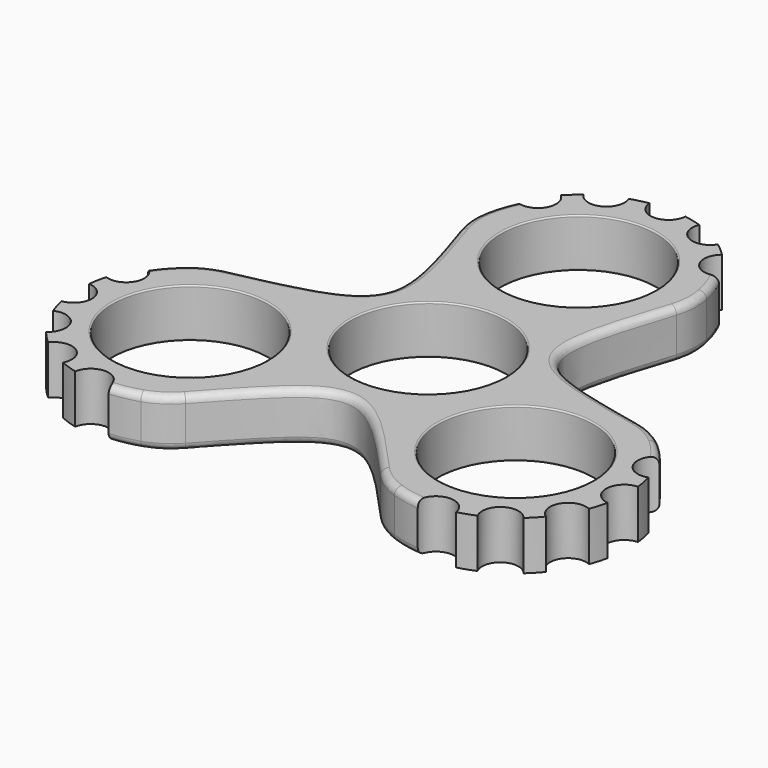
from build123d import *

# Parameters (mm, degrees)
F0_R     = 11.15
F2_DEPTH = 7
F3_COUNT = 3
F4_R     = 10
F5_R     = 1
F6_R     = 0.2


with BuildPart() as f2:
    # F0 (on Top) → F2 (new body)
    with BuildSketch(Plane.XY):
        with BuildLine():
            add(Edge.make_bspline(
                [(16.15, 27), (9.1228665673, 5.2670894684), (9.1238828606, 5.2676762256), (31.4576859022, 0.4863102711)],
                knots=[0, 0, 0, 0, 30.6153718044, 30.6153718044, 30.6153718044, 30.6153718044], degree=3))
            ThreePointArc((16.15, 27), (15.743464838, 30.6008075335), (14.544326329, 34.0203327297))
            ThreePointArc((14.544326329, 34.0203327297), (11.0995102001, 34.7719607126), (11.5714074372, 38.2661009192))
            ThreePointArc((11.5714074372, 38.2661009192), (10.6484349139, 39.1422128908), (9.6593461127, 39.9429336966))
            ThreePointArc((9.6593461127, 39.9429336966), (6.2566937093, 39.0189967896), (5.0618572759, 42.3362349004))
            ThreePointArc((5.0618572759, 42.3362349004), (3.8386271611, 42.6871744275), (2.5915629578, 42.9407120743))
            ThreePointArc((2.5915629578, 42.9407120743), (0, 40.55), (-2.5915629578, 42.9407120743))
            ThreePointArc((-2.5915629578, 42.9407120743), (-3.8386271611, 42.6871744275), (-5.0618572759, 42.3362349004))
            ThreePointArc((-5.0618572759, 42.3362349004), (-4.9089077714, 41.8409790869), (-4.8572401037, 41.3252249558))
            ThreePointArc((-4.8572401037, 41.3252249558), (-6.7380306848, 38.8266778157), (-9.6593461127, 39.9429336966))
            ThreePointArc((-9.6593461127, 39.9429336966), (-10.6484349139, 39.1422128908), (-11.5714074372, 38.2661009192))
            ThreePointArc((-11.5714074372, 38.2661009192), (-10.8765905938, 37.3699357767), (-10.6293055153, 36.2632594471))
            ThreePointArc((-10.6293055153, 36.2632594471), (-11.9368377431, 34.0072614289), (-14.544326329, 34.0203327297))
            ThreePointArc((-14.544326329, 34.0203327297), (-15.743464838, 30.6008075335), (-16.15, 27))
            Line((-16.15, 27), (-9.1757083535, 9.2008290812))
            Line((-9.1757083535, 9.2008290812), (-13.4726099074, 2.1395626913))
            Line((-13.4726099074, 2.1395626913), (-31.4576859022, 0.4863102711))
            ThreePointArc((-31.4576859022, 0.4863102711), (-34.3728091194, -1.6661632734), (-36.7346355536, -4.414410283))
            ThreePointArc((-36.7346355536, -4.414410283), (-35.7722477295, -5.3671973644), (-35.4195566628, -6.6747150729))
            ThreePointArc((-35.4195566628, -6.6747150729), (-36.5353839378, -8.8094823488), (-38.9251192184, -9.1119176615))
            ThreePointArc((-38.9251192184, -9.1119176615), (-39.2223681807, -10.3492912994), (-39.4212683393, -11.6062277308))
            ThreePointArc((-39.4212683393, -11.6062277308), (-37.6451874832, -12.4002525195), (-36.9173146807, -14.204453106))
            ThreePointArc((-36.9173146807, -14.204453106), (-37.5682712092, -15.9252754518), (-39.1951835622, -16.7844204589))
            ThreePointArc((-39.1951835622, -16.7844204589), (-38.8874910505, -18.0192385766), (-38.4835289918, -19.2259966802))
            ThreePointArc((-38.4835289918, -19.2259966802), (-35.9793532926, -19.3775258445), (-34.7689961733, -21.575))
            ThreePointArc((-34.7689961733, -21.575), (-35.0667930587, -22.7832470025), (-35.891966034, -23.7147153941))
            ThreePointArc((-35.891966034, -23.7147153941), (-35.0488638894, -24.6679358509), (-34.1333262864, -25.5518144414))
            ThreePointArc((-34.1333262864, -25.5518144414), (-31.2325645904, -24.6559742472), (-29.460074577, -27.1207718499))
            ThreePointArc((-29.460074577, -27.1207718499), (-29.5366645716, -27.7471917925), (-29.7619222266, -28.3367059659))
            ThreePointArc((-29.7619222266, -28.3367059659), (-28.5739332668, -28.7929215913), (-27.3537117813, -29.1541832578))
            ThreePointArc((-27.3537117813, -29.1541832578), (-24.572303502, -26.9976953196), (-22.1902511476, -29.5885443742))
            ThreePointArc((-22.1902511476, -29.5885443742), (-22.1902656669, -29.597233459), (-22.1903092246, -29.6059224467))
            ThreePointArc((-22.1903092246, -29.6059224467), (-18.6293442813, -28.9346442601), (-15.3076859022, -27.4863102711))
            Line((-15.3076859022, -27.4863102711), (-3.012867426, -11.4551726729))
            Line((-3.012867426, -11.4551726729), (3.3642563503, -11.4551726729))
            Line((3.3642563503, -11.4551726729), (15.3076859022, -27.4863102711))
            ThreePointArc((15.3076859022, -27.4863102711), (18.6293442813, -28.9346442601), (22.1903092246, -29.6059224467))
            ThreePointArc((22.1903092246, -29.6059224467), (24.5636462164, -26.9984381591), (27.3537117813, -29.1541832578))
            ThreePointArc((27.3537117813, -29.1541832578), (28.5739332668, -28.7929215913), (29.7619222266, -28.3367059659))
            ThreePointArc((29.7619222266, -28.3367059659), (30.6630955953, -24.9279540908), (34.1333262864, -25.5518144414))
            ThreePointArc((34.1333262864, -25.5518144414), (35.0488638894, -24.6679358509), (35.891966034, -23.7147153941))
            ThreePointArc((35.891966034, -23.7147153941), (35.1173301235, -20.275), (38.4835289918, -19.2259966802))
            ThreePointArc((38.4835289918, -19.2259966802), (38.8874910505, -18.0192385766), (39.1951835622, -16.7844204589))
            ThreePointArc((39.1951835622, -16.7844204589), (36.9197893046, -14.0910426988), (39.4212683393, -11.6062277308))
            ThreePointArc((39.4212683393, -11.6062277308), (39.2223681807, -10.3492912994), (38.9251192184, -9.1119176615))
            ThreePointArc((38.9251192184, -9.1119176615), (35.6631564165, -7.7735225534), (36.7346355536, -4.414410283))
            ThreePointArc((36.7346355536, -4.414410283), (34.3728091194, -1.6661632734), (31.4576859022, 0.4863102711))
        make_face()
        with Locations((-23.3826859022, -13.5)):
            Circle(F0_R, mode=Mode.SUBTRACT)
        with Locations((23.3826859022, -13.5)):
            Circle(F0_R, mode=Mode.SUBTRACT)
        Circle(F0_R, mode=Mode.SUBTRACT)
        with Locations((0, 27)):
            Circle(F0_R, mode=Mode.SUBTRACT)
    extrude(amount=F2_DEPTH)

    # F3: F2 ×3 about axis
    f3_axis = Axis((0, 0, 0.0969832763), (0, 0, -1))


with BuildPart() as f2_1:
    add(f2.part)
    for i in range(1, F3_COUNT):
        add(f2.part.rotate(f3_axis, i * 360 / F3_COUNT))

    # F4
    f4_edges = [f2_1.edges().sort_by_distance(p)[0] for p in [
        (16.15, 27, 3.5),
        (31.457686, 0.48631, 3.5),
        (15.307686, -27.48631, 3.5),
        (-15.307686, -27.48631, 3.5),
        (-31.457686, 0.48631, 3.5),
        (-16.15, 27, 3.5),
    ]]
    fillet(f4_edges, radius=F4_R)

    # F5
    f5_edges = [f2_1.edges().sort_by_distance(p)[0] for p in [
        (12.792368, 7.388272, 7),
        (-12.794616, 7.38438, 7),
        (0.002247, -14.772652, 7),
        (0.002247, -14.772652, 0),
        (-12.794616, 7.38438, 0),
        (12.792368, 7.388272, 0),
        (15.312256, 32.133938, 7),
        (16.014291, 27.63337, 7),
        (31.938289, 0.052164, 7),
        (35.484822, -2.806039, 7),
        (-15.31231, 32.133776, 7),
        (-16.01432, 27.633287, 7),
        (-31.938346, 0.052098, 7),
        (20.172679, -29.327772, 7),
        (-35.484935, -2.806167, 7),
        (15.924055, -27.685468, 7),
        (-15.923969, -27.685451, 7),
        (-20.172512, -29.327738, 7),
        (15.312256, 32.133938, 0),
        (16.014291, 27.63337, 0),
        (31.938289, 0.052164, 0),
        (35.484822, -2.806039, 0),
        (-15.31231, 32.133776, 0),
        (-16.01432, 27.633287, 0),
        (-31.938346, 0.052098, 0),
        (20.172679, -29.327772, 0),
        (-35.484935, -2.806167, 0),
        (15.924055, -27.685468, 0),
        (-15.923969, -27.685451, 0),
        (-20.172512, -29.327738, 0),
    ]]
    fillet(f5_edges, radius=F5_R)

    # F6
    f6_edges = [f2_1.edges().sort_by_distance(p)[0] for p in [
        (-11.15, 0, 0),
        (11.15, 0, 3.5),
        (-11.15, 0, 7),
        (12.232686, -13.5, 0),
        (34.532686, -13.5, 3.5),
        (12.232686, -13.5, 7),
        (-34.532686, -13.5, 0),
        (-12.232686, -13.5, 3.5),
        (-34.532686, -13.5, 7),
        (-11.15, 27, 0),
        (11.15, 27, 3.5),
        (-11.15, 27, 7),
    ]]
    fillet(f6_edges, radius=F6_R)


solid = f2_1.part
